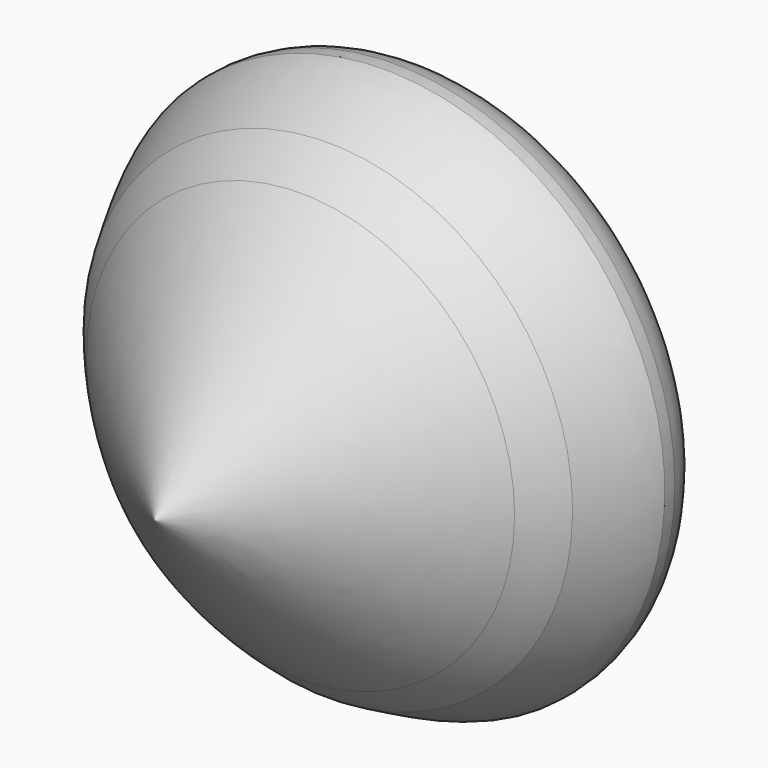
from build123d import *


with BuildPart() as f1:
    # F0 (on Top) → F1 (revolve)
    with BuildSketch(Plane.XY):
        with BuildLine():
            Line((0, -77.1725550294), (0, -10.2951908484))
            add(Edge.make_bspline(
                [(-42.6886081696, -31.1840437353), (-41.9741262251, -26.3481394016), (-31.6279975873, -19.2652491052), (-28.4993753923, -33.9943389303), (0.3572648065, -37.670465576), (-9.2300311467, -9.4699013844), (-2.4061661468, -10.0800470923), (0, -10.2951908484)],
                knots=[0.3053795427, 0.3053795427, 0.3053795427, 0.3053795427, 0.4389974584, 0.5677136643, 0.7354119084, 0.9067034725, 1, 1, 1, 1], degree=3))
            add(Edge.make_bspline(
                [(-42.7384666865, -33.156890188), (-42.7977850628, -32.4787986109), (-42.7826820789, -31.8207742077), (-42.6886081696, -31.1840437353)],
                knots=[0.2877864324, 0.2877864324, 0.2877864324, 0.2877864324, 0.3053795427, 0.3053795427, 0.3053795427, 0.3053795427], degree=3))
            add(Edge.make_bspline(
                [(-37.354488354, -44.0324225911), (-39.7064828767, -39.8275234586), (-42.0563257906, -35.6210082892), (-42.7384666865, -33.156890188)],
                knots=[0, 0, 0, 0, 0.3852866289, 0.3852866289, 0.3852866289, 0.3852866289], degree=3))
            add(Edge.make_bspline(
                [(-32.7153271789, -49.3045997466), (-34.4531037106, -47.4956005938), (-36.0120744387, -45.7348151143), (-37.354488354, -44.0324225911)],
                knots=[0.1687000542, 0.1687000542, 0.1687000542, 0.1687000542, 0.2043174512, 0.2043174512, 0.2043174512, 0.2043174512], degree=3))
            add(Edge.make_bspline(
                [(0, -77.1725550294), (-12.2422169317, -67.5226952717), (-24.4844338634, -57.8728355141), (-32.7153271789, -49.3045997466)],
                knots=[0, 0, 0, 0, 0.1687000542, 0.1687000542, 0.1687000542, 0.1687000542], degree=3))
        make_face()
    revolve(axis=Axis((0, -1.2533664703, 0), (0, -1, 0)))


solid = f1.part
